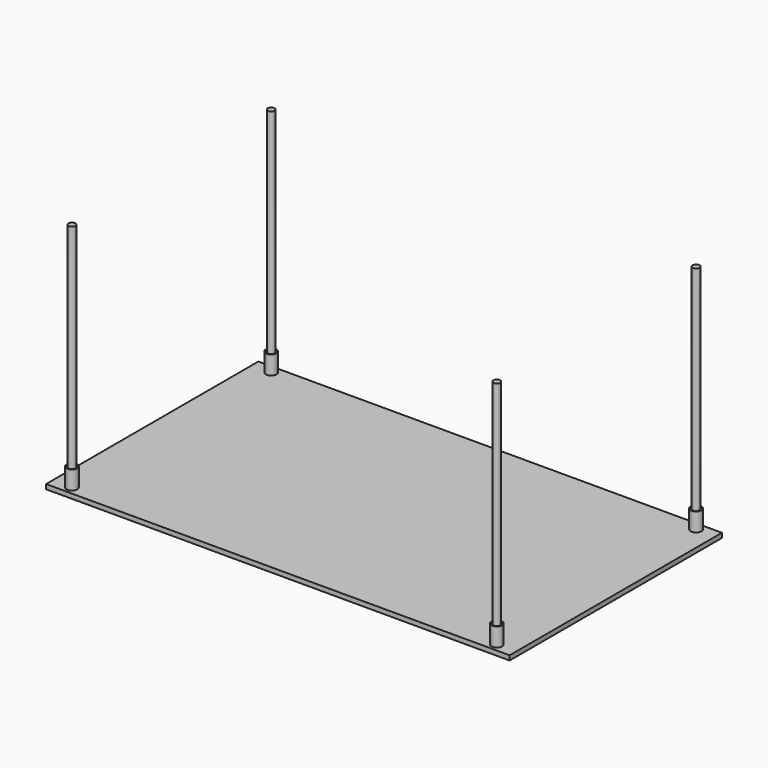
from build123d import *

# Parameters (mm, degrees)
F0_W     = 100.1612991095
F0_H     = 57.3387145996
F1_DEPTH = 1
F4_R     = 0.75
F5_DEPTH = 50
F6_R     = 1.159755705
F6_R_2   = 0.9527404517
F7_DEPTH = 5


# Not quite as in the source:
# - a feature names something its author has since deleted; it is built from what else it names


with BuildPart() as f1:
    # F0 (on Top) → F1 (new body)
    with BuildSketch(Plane.XY):
        Rectangle(F0_W, F0_H)
    extrude(amount=F1_DEPTH)

    # F4 (on face) → F5 (join)
    with BuildSketch(Plane.XY.offset(1)):
        with Locations((-45.9097400308, 26.9193572998)):
            Circle(F4_R)
    extrude(amount=F5_DEPTH)

    # F6 (on Top) → F7 (join)
    with BuildSketch(Plane.XY):
        with Locations((-45.9088794887, 26.9124545157)):
            Circle(F6_R)
        with Locations((-45.9088794887, 26.9124545157)):
            Circle(F6_R_2, mode=Mode.SUBTRACT)
    extrude(amount=F7_DEPTH)

    # F8: F1 across plane


with BuildPart() as f1_1:
    add(f1.part)
    add(f1.part.mirror(Plane.XZ))

    # F9: F1 across plane


with BuildPart() as f1_2:
    add(f1_1.part)
    add(f1_1.part.mirror(Plane.YZ))


solid = f1_2.part
